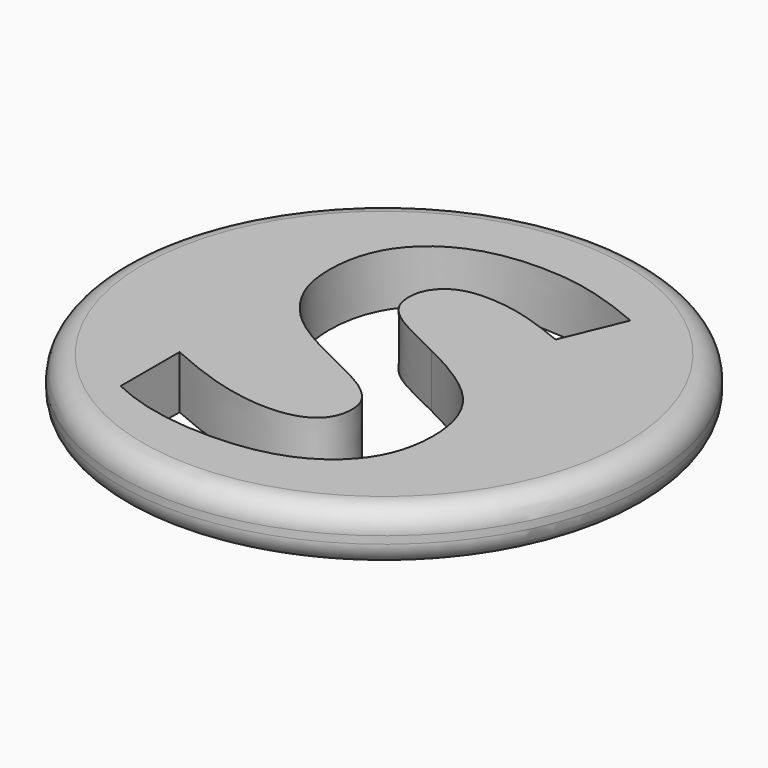
from build123d import *

# Parameters (mm, degrees)
F0_R         = 11.605
F1_DEPTH     = 1.165
F2_R         = 1
F3_TEXT_SIZE = 23.001632628
F4_DEPTH     = 2.331


# Not quite as in the source:
# - Text() gives the source's letters only with a copy of the font that has no kerning and outlines rounded to 1/6400 em; it was checked with that copy


with BuildPart() as f1:
    # F0 (on Top) → F1 (new body, symmetric)
    with BuildSketch(Plane.XY):
        Circle(F0_R)
    extrude(amount=F1_DEPTH, both=True)

    # F2
    f2_edges = [f1.edges().sort_by_distance(p)[0] for p in [
        (-11.605, 0, 1.165),
        (-11.605, 0, -1.165),
    ]]
    fillet(f2_edges, radius=F2_R)

    # F3 (on face) → F4 (cut, through all)
    with BuildSketch(Plane.XY.offset(1.165)):
        with Locations((-6.6255483984, -8.2805877461)):
            Text('S', F3_TEXT_SIZE, font='Open Sans', font_style=FontStyle.BOLD, text_align=(TextAlign.LEFT, TextAlign.BOTTOM))
    extrude(amount=-F4_DEPTH, mode=Mode.SUBTRACT)


solid = f1.part
